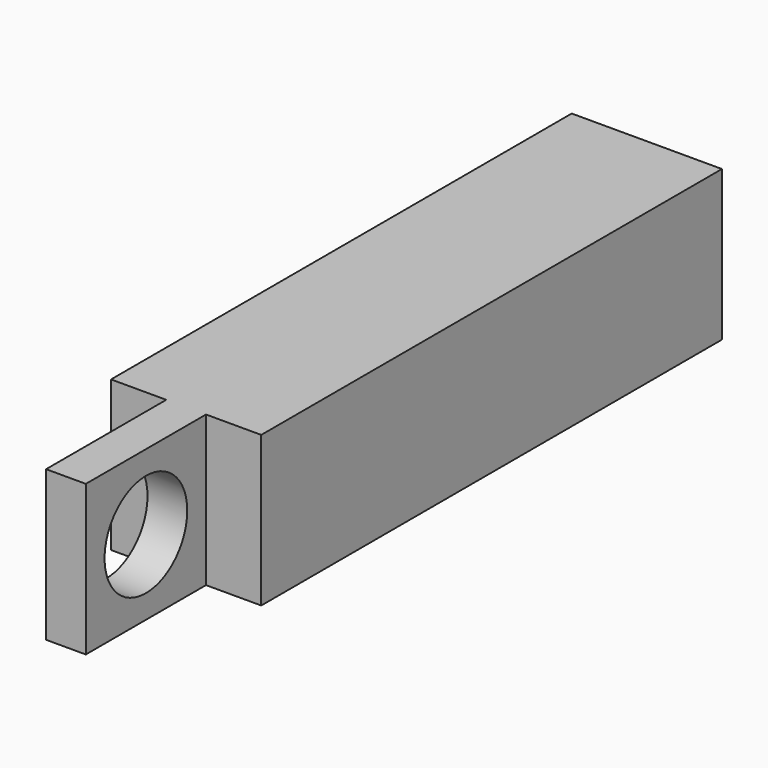
from build123d import *

# Parameters (mm, degrees)
F0_W     = 30
F0_H     = 30
F0_R     = 10.31875
F1_DEPTH = 3.96875
F0_W_2   = 115
F2_DEPTH = 15


# Not quite as in the source:
# - a length typed as a fraction of an inch, garbled in the dataset ("3 / 203.2 mm" for 3/8 in), is restored


with BuildPart() as f1:
    # F0 (on Right) → F1 (new body, symmetric)
    with BuildSketch(Plane.YZ):
        Rectangle(F0_W, F0_H)
        Circle(F0_R, mode=Mode.SUBTRACT)
    extrude(amount=F1_DEPTH, both=True)

    # F0 (on Right) → F2 (join, symmetric)
    with BuildSketch(Plane.YZ):
        with Locations((72.5, 0)):
            Rectangle(F0_W_2, F0_H)
    extrude(amount=F2_DEPTH, both=True)


solid = f1.part
